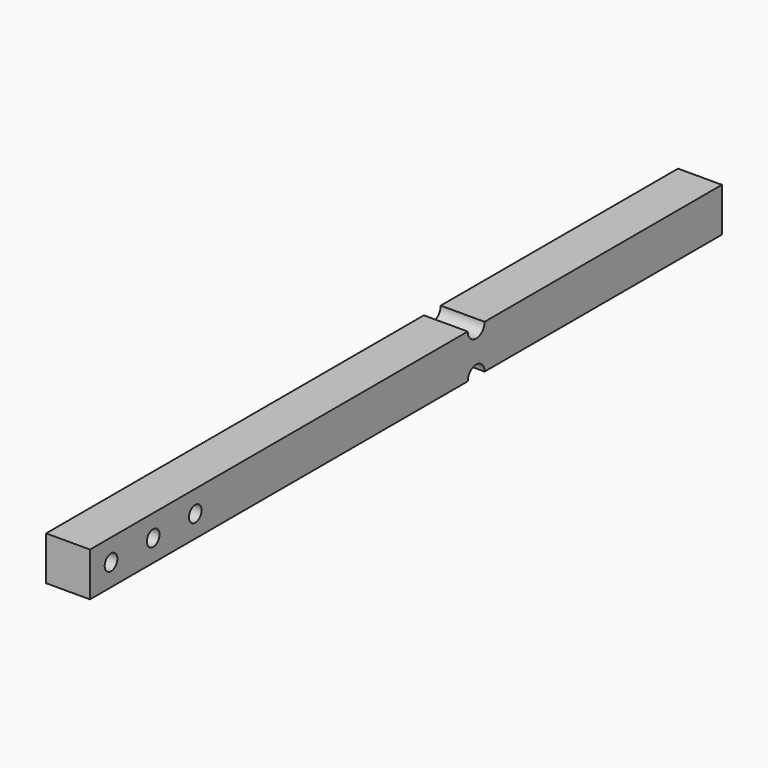
from build123d import *

# Parameters (mm, degrees)
F0_W          = 350
F0_H          = 25
F1_DEPTH      = 12.5
F1_DEPTH_BACK = 12.5
F3_DEPTH      = 25
F5_DEPTH      = 100
F7_D          = 9


# Not quite as in the source:
# - a pattern or mirror of a feature is missing from the dataset's text; its kind, count and spacing are read off the source's solid


with BuildPart() as f1:
    # F0 (on Right) → F1 (new body, two sides)
    with BuildSketch(Plane.YZ) as f1_sk:
        with Locations((175, 12.5)):
            Rectangle(F0_W, F0_H)
    extrude(amount=F1_DEPTH)
    extrude(f1_sk.sketch, amount=-F1_DEPTH_BACK)

    # F2 (on face) → F3 (cut)
    with BuildSketch(Plane.YZ.offset(12.5)):
        with BuildLine():
            ThreePointArc((169, 25), (175, 19), (181, 25))
            Line((181, 25), (169, 25))
        make_face()
    f3 = extrude(amount=-F3_DEPTH, mode=Mode.SUBTRACT)

    # F3_copies: F3 across plane
    add(f3.mirror(Plane(origin=(0, 0, 12.5), x_dir=(-1, 0, 0), z_dir=(0, 0, -1))), mode=Mode.SUBTRACT)

    # F5 (add): a face of the model
    f5_faces = [f1.faces().sort_by_distance(p)[0] for p in [
        (0, 0, 12.5),
    ]]
    extrude(f5_faces, amount=F5_DEPTH)

    # F7 (through all)
    with Locations(Plane.YZ.offset(12.5)):
        with Locations((-85, 12.5), (-55, 12.5), (-25, 12.5)):
            Hole(F7_D / 2)


solid = f1.part
